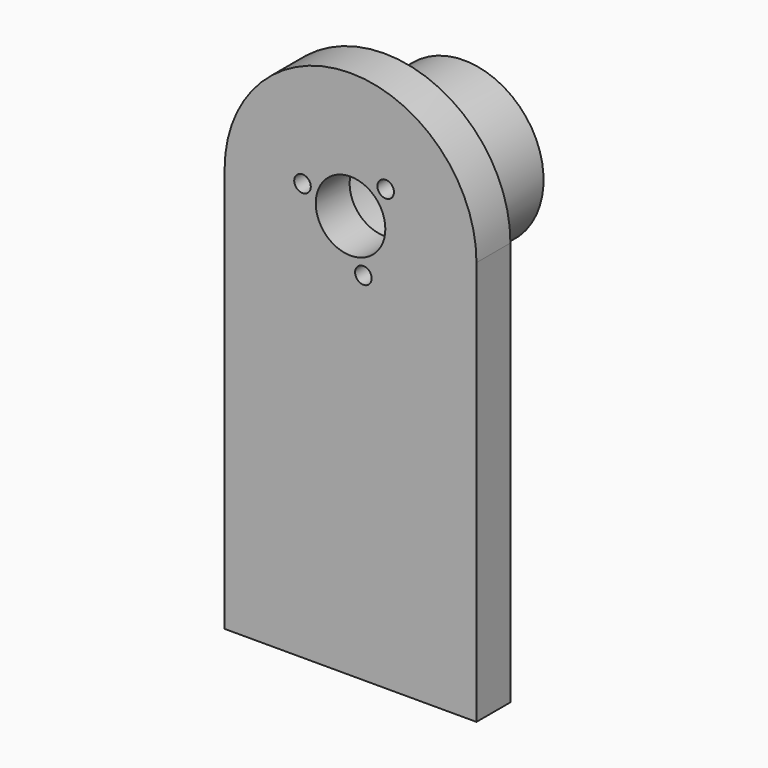
from build123d import *

# Parameters (mm, degrees)
F1_DEPTH        = 6.4
F2_R            = 1.25
F3_DEPTH        = 6.401
F3_COPIES_COUNT = 3
F4_R            = 5.25
F5_DEPTH        = 6.401
F6_R            = 12
F6_R_2          = 10
F7_DEPTH        = 15


# Not quite as in the source:
# - a pattern or mirror of a feature is missing from the dataset's text; its kind, count and spacing are read off the source's solid


with BuildPart() as f1:
    # F0 (on Front) → F1 (new body)
    with BuildSketch(Plane.XZ):
        with BuildLine():
            Line((-19, 0), (-19, -61))
            Line((-19, -61), (19, -61))
            Line((19, -61), (19, 0))
            ThreePointArc((19, 0), (0, 19), (-19, 0))
        make_face()
    extrude(amount=F1_DEPTH)

    # F2 (on Front) → F3 (cut, through all)
    with BuildSketch(Plane.XZ):
        with Locations((5.3033008589, 5.3033008589)):
            Circle(F2_R)
    f3 = extrude(amount=F3_DEPTH, mode=Mode.SUBTRACT)

    # F3_copies: F3 ×3 about axis
    f3_copies_axis = Axis((0, 0, 0), (0, 1, 0))
    for i in range(1, F3_COPIES_COUNT):
        add(f3.rotate(f3_copies_axis, i * 360 / F3_COPIES_COUNT), mode=Mode.SUBTRACT)

    # F4 (on Front) → F5 (cut, through all)
    with BuildSketch(Plane.XZ):
        Circle(F4_R)
    extrude(amount=F5_DEPTH, mode=Mode.SUBTRACT)

    # F6 (on face) → F7 (join)
    with BuildSketch(Plane(origin=(0, 0, 0), x_dir=(-1, 0, 0), z_dir=(0, 1, 0))):
        Circle(F6_R)
        Circle(F6_R_2, mode=Mode.SUBTRACT)
    extrude(amount=F7_DEPTH)


solid = f1.part
